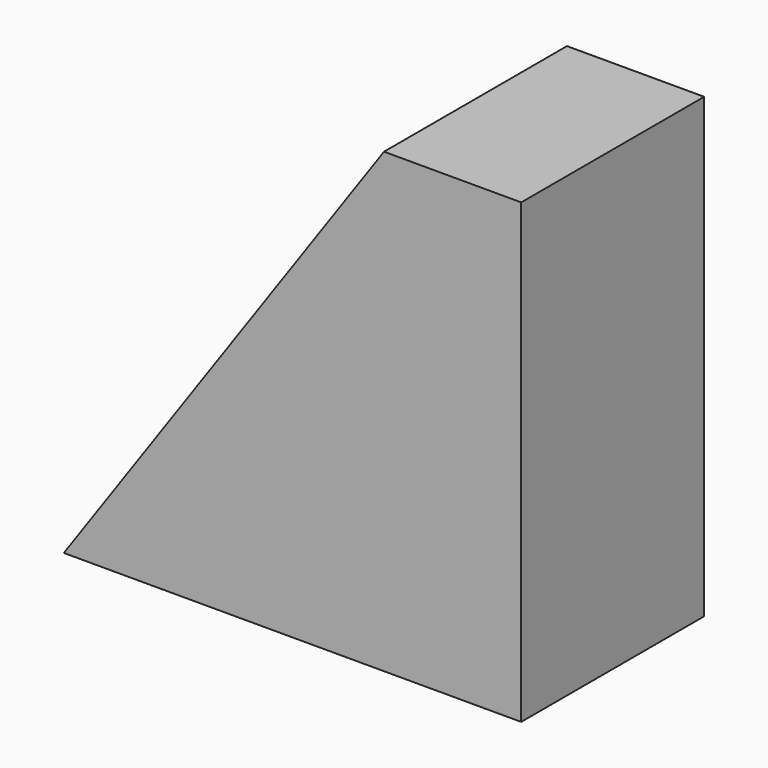
from build123d import *

# Parameters (mm, degrees)
F0_W     = 100
F0_H     = 100
F1_DEPTH = 50
F2_SIZE2 = 69.99999
F2_SIZE  = 99.99999


# Not quite as in the source:
# - a fillet or chamfer is up to 0.001 mm smaller than in the source, because OpenCascade refuses the exact size


with BuildPart() as f1:
    # F0 (on Front) → F1 (new body)
    with BuildSketch(Plane.XZ):
        with Locations((-50, 50)):
            Rectangle(F0_W, F0_H)
    extrude(amount=F1_DEPTH)

    # F2 (size 100 and 70 in the source; OpenCascade refuses exactly that, so slightly less here)
    f2_edges = [f1.edges().sort_by_distance(p)[0] for p in [
        (-100, -25, 100),
    ]]
    f2_side = f1.faces().sort_by_distance((-100, -25, 50))[0]
    chamfer(f2_edges, length=F2_SIZE, length2=F2_SIZE2, reference=f2_side)


solid = f1.part
